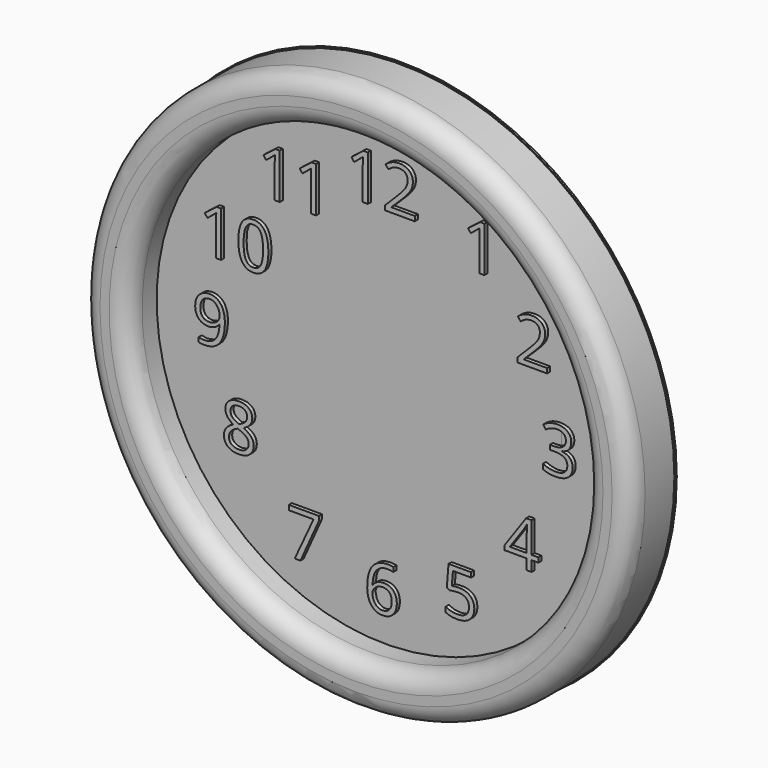
from build123d import *

# Parameters (mm, degrees)
F0_R         = 38.1
F0_R_2       = 31.75
F1_DEPTH     = 7.62
F2_DEPTH     = 2.54
F3_DEPTH     = 2.54
F4_DEPTH     = 2.54
F5_DEPTH     = 2.54
F0_TEXT_SIZE = 8.8194444444
F6_DEPTH     = 3.0734
F7_R         = 2.54
F8_DEPTH     = 2.54
F9_DEPTH     = 2.54
F10_R        = 38.2366779264
F11_DEPTH    = 0.254


# Not quite as in the source:
# - Text() gives the source's letters only with a copy of the font that has no kerning and outlines rounded to 1/6400 em; it was checked with that copy


with BuildPart() as f1:
    # F0 (on Front) → F1 (new body)
    with BuildSketch(Plane.XZ):
        Circle(F0_R)
        Circle(F0_R_2, mode=Mode.SUBTRACT)
    extrude(amount=F1_DEPTH)

    # F7
    f7_edges = [f1.edges().sort_by_distance(p)[0] for p in [
        (-38.1, -7.62, 0),
        (-31.75, -7.62, 0),
    ]]
    fillet(f7_edges, radius=F7_R)


with BuildPart() as f2:
    # F0 (on Front) → F2 (new body)
    with BuildSketch(Plane.XZ):
        with BuildLine():
            add(Edge.make_bspline(
                [(-18.9333114864, 13.2705580962), (-19.256461443, 12.6483738514), (-19.256461443, 11.2744697715)],
                knots=[0, 0, 0, 1, 1, 1], degree=2))
            add(Edge.make_bspline(
                [(-19.256461443, 11.2744697715), (-19.256461443, 9.9005656917), (-18.9333114864, 9.2735583132)],
                knots=[0, 0, 0, 1, 1, 1], degree=2))
            add(Edge.make_bspline(
                [(-18.9333114864, 9.2735583132), (-18.6101615298, 8.6465509347), (-17.9046059742, 8.6465509347)],
                knots=[0, 0, 0, 1, 1, 1], degree=2))
            add(Edge.make_bspline(
                [(-17.9046059742, 8.6465509347), (-17.1894041513, 8.6465509347), (-16.8690102711, 9.2818265424)],
                knots=[0, 0, 0, 1, 1, 1], degree=2))
            add(Edge.make_bspline(
                [(-16.8690102711, 9.2818265424), (-16.5486163909, 9.91710215), (-16.5486163909, 11.2744697715)],
                knots=[0, 0, 0, 1, 1, 1], degree=2))
            add(Edge.make_bspline(
                [(-16.5486163909, 11.2744697715), (-16.5486163909, 12.6304593549), (-16.8690102711, 13.2616008479)],
                knots=[0, 0, 0, 1, 1, 1], degree=2))
            add(Edge.make_bspline(
                [(-16.8690102711, 13.2616008479), (-17.1894041513, 13.892742341), (-17.9046059742, 13.892742341)],
                knots=[0, 0, 0, 1, 1, 1], degree=2))
            add(Edge.make_bspline(
                [(-17.9046059742, 13.892742341), (-18.6101615298, 13.892742341), (-18.9333114864, 13.2705580962)],
                knots=[0, 0, 0, 1, 1, 1], degree=2))
        make_face()
    extrude(amount=F2_DEPTH)


with BuildPart() as f3:
    # F0 (on Front) → F3 (new body)
    with BuildSketch(Plane.XZ):
        with BuildLine():
            Line((17.7058799275, -13.9019929305), (20.0526789726, -13.9019929305))
            Line((20.0526789726, -13.9019929305), (20.0526789726, -11.8087529131))
            add(Edge.make_bspline(
                [(20.0526789726, -11.8087529131), (20.0526789726, -11.1927698402), (20.0967761949, -10.4183123749)],
                knots=[0, 0, 0, 1, 1, 1], degree=2))
            Line((20.0967761949, -10.4183123749), (20.06232524, -10.4183123749))
            add(Edge.make_bspline(
                [(20.06232524, -10.4183123749), (19.8556195108, -10.8317238333), (19.6737184692, -11.1031973576)],
                knots=[0, 0, 0, 1, 1, 1], degree=2))
            Line((19.6737184692, -11.1031973576), (17.7058799275, -13.9019929305))
        make_face()
    extrude(amount=F3_DEPTH)


with BuildPart() as f4:
    # F0 (on Front) → F4 (new body)
    with BuildSketch(Plane.XZ):
        with BuildLine():
            add(Edge.make_bspline(
                [(-23.2508578055, 2.622299725), (-23.5671175712, 2.842096817), (-23.9763949149, 2.842096817)],
                knots=[0, 0, 0, 1, 1, 1], degree=2))
            add(Edge.make_bspline(
                [(-23.9763949149, 2.842096817), (-24.5923779878, 2.842096817), (-24.9279302882, 2.4459108361)],
                knots=[0, 0, 0, 1, 1, 1], degree=2))
            add(Edge.make_bspline(
                [(-24.9279302882, 2.4459108361), (-25.2634825885, 2.0497248552), (-25.2634825885, 1.3427912614)],
                knots=[0, 0, 0, 1, 1, 1], degree=2))
            add(Edge.make_bspline(
                [(-25.2634825885, 1.3427912614), (-25.2634825885, 0.7226740739), (-24.9534239948, 0.3678292389)],
                knots=[0, 0, 0, 1, 1, 1], degree=2))
            add(Edge.make_bspline(
                [(-24.9534239948, 0.3678292389), (-24.643365401, 0.0129844038), (-24.0108458698, 0.0129844038)],
                knots=[0, 0, 0, 1, 1, 1], degree=2))
            add(Edge.make_bspline(
                [(-24.0108458698, 0.0129844038), (-23.6181049844, 0.0129844038), (-23.2887538559, 0.1721478153)],
                knots=[0, 0, 0, 1, 1, 1], degree=2))
            add(Edge.make_bspline(
                [(-23.2887538559, 0.1721478153), (-22.9594027274, 0.3313112267), (-22.7699224757, 0.6069188656)],
                knots=[0, 0, 0, 1, 1, 1], degree=2))
            add(Edge.make_bspline(
                [(-22.7699224757, 0.6069188656), (-22.5804422239, 0.8825265045), (-22.5804422239, 1.1843168691)],
                knots=[0, 0, 0, 1, 1, 1], degree=2))
            add(Edge.make_bspline(
                [(-22.5804422239, 1.1843168691), (-22.5804422239, 1.6363133969), (-22.7575201319, 2.0194080149)],
                knots=[0, 0, 0, 1, 1, 1], degree=2))
            add(Edge.make_bspline(
                [(-22.7575201319, 2.0194080149), (-22.9345980399, 2.402502633), (-23.2508578055, 2.622299725)],
                knots=[0, 0, 0, 1, 1, 1], degree=2))
        make_face()
    extrude(amount=F4_DEPTH)


with BuildPart() as f5:
    # F0 (on Front) → F5 (new body)
    with BuildSketch(Plane.XZ):
        with BuildLine():
            add(Edge.make_bspline(
                [(-0.6952202691, -27.1951703559), (-0.3789605035, -27.4191015625), (0.0261827257, -27.4191015625)],
                knots=[0, 0, 0, 1, 1, 1], degree=2))
            add(Edge.make_bspline(
                [(0.0261827257, -27.4191015625), (0.638031684, -27.4191015625), (0.9756510417, -27.0332508681)],
                knots=[0, 0, 0, 1, 1, 1], degree=2))
            add(Edge.make_bspline(
                [(0.9756510417, -27.0332508681), (1.3132703993, -26.6474001736), (1.3132703993, -25.9197960069)],
                knots=[0, 0, 0, 1, 1, 1], degree=2))
            add(Edge.make_bspline(
                [(1.3132703993, -25.9197960069), (1.3132703993, -25.2955447049), (0.999077691, -24.9379437934)],
                knots=[0, 0, 0, 1, 1, 1], degree=2))
            add(Edge.make_bspline(
                [(0.999077691, -24.9379437934), (0.6848849826, -24.5803428819), (0.0606336806, -24.5803428819)],
                knots=[0, 0, 0, 1, 1, 1], degree=2))
            add(Edge.make_bspline(
                [(0.0606336806, -24.5803428819), (-0.3265950521, -24.5803428819), (-0.6497450087, -24.7401953125)],
                knots=[0, 0, 0, 1, 1, 1], degree=2))
            add(Edge.make_bspline(
                [(-0.6497450087, -24.7401953125), (-0.9728949653, -24.9000477431), (-1.1644422743, -25.1797894965)],
                knots=[0, 0, 0, 1, 1, 1], degree=2))
            add(Edge.make_bspline(
                [(-1.1644422743, -25.1797894965), (-1.3559895833, -25.45953125), (-1.3559895833, -25.7613216146)],
                knots=[0, 0, 0, 1, 1, 1], degree=2))
            add(Edge.make_bspline(
                [(-1.3559895833, -25.7613216146), (-1.3559895833, -26.2050499132), (-1.183734809, -26.5881445313)],
                knots=[0, 0, 0, 1, 1, 1], degree=2))
            add(Edge.make_bspline(
                [(-1.183734809, -26.5881445313), (-1.0114800347, -26.9712391493), (-0.6952202691, -27.1951703559)],
                knots=[0, 0, 0, 1, 1, 1], degree=2))
        make_face()
    extrude(amount=F5_DEPTH)


with BuildPart() as f5b:
    # F0 (on Front) → F5, piece 2 (new body)
    with BuildSketch(Plane.XZ):
        with BuildLine():
            add(Edge.make_bspline(
                [(-20.990759851, -12.3462794049), (-21.2787698337, -12.679764648), (-21.2787698337, -13.1455415577)],
                knots=[0, 0, 0, 1, 1, 1], degree=2))
            add(Edge.make_bspline(
                [(-21.2787698337, -13.1455415577), (-21.2787698337, -13.6623058806), (-20.919790884, -13.9510048824)],
                knots=[0, 0, 0, 1, 1, 1], degree=2))
            add(Edge.make_bspline(
                [(-20.919790884, -13.9510048824), (-20.5608119344, -14.2397038841), (-19.9103779066, -14.2397038841)],
                knots=[0, 0, 0, 1, 1, 1], degree=2))
            add(Edge.make_bspline(
                [(-19.9103779066, -14.2397038841), (-19.268212108, -14.2397038841), (-18.9106111965, -13.9379135195)],
                knots=[0, 0, 0, 1, 1, 1], degree=2))
            add(Edge.make_bspline(
                [(-18.9106111965, -13.9379135195), (-18.553010285, -13.6361231549), (-18.553010285, -13.1110906028)],
                knots=[0, 0, 0, 1, 1, 1], degree=2))
            add(Edge.make_bspline(
                [(-18.553010285, -13.1110906028), (-18.553010285, -12.6935450299), (-18.8892516045, -12.368328016)],
                knots=[0, 0, 0, 1, 1, 1], degree=2))
            add(Edge.make_bspline(
                [(-18.8892516045, -12.368328016), (-19.2254929239, -12.0431110021), (-20.0605840698, -11.737186523)],
                knots=[0, 0, 0, 1, 1, 1], degree=2))
            add(Edge.make_bspline(
                [(-20.0605840698, -11.737186523), (-20.7027498684, -12.0127941619), (-20.990759851, -12.3462794049)],
                knots=[0, 0, 0, 1, 1, 1], degree=2))
        make_face()
    extrude(amount=F5_DEPTH)


with BuildPart() as f5c:
    # F0 (on Front) → F5, piece 3 (new body)
    with BuildSketch(Plane.XZ):
        with BuildLine():
            add(Edge.make_bspline(
                [(-19.0677075507, -9.1850597869), (-19.3798332017, -8.9287446827), (-19.9269143649, -8.9287446827)],
                knots=[0, 0, 0, 1, 1, 1], degree=2))
            add(Edge.make_bspline(
                [(-19.9269143649, -8.9287446827), (-20.4657272989, -8.9287446827), (-20.7716517781, -9.1871268442)],
                knots=[0, 0, 0, 1, 1, 1], degree=2))
            add(Edge.make_bspline(
                [(-20.7716517781, -9.1871268442), (-21.0775762573, -9.4455090056), (-21.0775762573, -9.8768349605)],
                knots=[0, 0, 0, 1, 1, 1], degree=2))
            add(Edge.make_bspline(
                [(-21.0775762573, -9.8768349605), (-21.0775762573, -10.2723319223), (-20.8233282104, -10.5568968094)],
                knots=[0, 0, 0, 1, 1, 1], degree=2))
            add(Edge.make_bspline(
                [(-20.8233282104, -10.5568968094), (-20.5690801635, -10.8414616966), (-19.8841951809, -11.1253375646)],
                knots=[0, 0, 0, 1, 1, 1], degree=2))
            add(Edge.make_bspline(
                [(-19.8841951809, -11.1253375646), (-19.268212108, -10.8676444223), (-19.0118970038, -10.5699881723)],
                knots=[0, 0, 0, 1, 1, 1], degree=2))
            add(Edge.make_bspline(
                [(-19.0118970038, -10.5699881723), (-18.7555818996, -10.2723319223), (-18.7555818996, -9.8768349605)],
                knots=[0, 0, 0, 1, 1, 1], degree=2))
            add(Edge.make_bspline(
                [(-18.7555818996, -9.8768349605), (-18.7555818996, -9.441374891), (-19.0677075507, -9.1850597869)],
                knots=[0, 0, 0, 1, 1, 1], degree=2))
        make_face()
    extrude(amount=F5_DEPTH)


with BuildPart() as f6:
    # F0 (on Front) → F6 (new body)
    with BuildSketch(Plane.XZ):
        with Locations((21.9082459122, -3.175)):
            Text('3', F0_TEXT_SIZE, font='Open Sans', text_align=(TextAlign.LEFT, TextAlign.BOTTOM))
        with Locations((16.8060209865, -15.9993670624)):
            Text('4', F0_TEXT_SIZE, font='Open Sans', text_align=(TextAlign.LEFT, TextAlign.BOTTOM))
        with Locations((8.2414952257, -25.0474884677)):
            Text('5', F0_TEXT_SIZE, font='Open Sans', text_align=(TextAlign.LEFT, TextAlign.BOTTOM))
        with Locations((-2.5920898438, -27.94)):
            Text('6', F0_TEXT_SIZE, font='Open Sans', text_align=(TextAlign.LEFT, TextAlign.BOTTOM))
        with Locations((-13.3781325955, -25.0474884677)):
            Text('7', F0_TEXT_SIZE, font='Open Sans', text_align=(TextAlign.LEFT, TextAlign.BOTTOM))
        with Locations((-22.4335658406, -14.7344195959)):
            Text('8', F0_TEXT_SIZE, font='Open Sans', text_align=(TextAlign.LEFT, TextAlign.BOTTOM))
        with Locations((-26.4265468246, -2.9332612559)):
            Text('9', F0_TEXT_SIZE, font='Open Sans', text_align=(TextAlign.LEFT, TextAlign.BOTTOM))
        with Locations((-25.4617674326, 8.117384268)):
            Text('10', F0_TEXT_SIZE, font='Open Sans', text_align=(TextAlign.LEFT, TextAlign.BOTTOM))
        with Locations((18.3173481208, 8.9695071709)):
            Text('2', F0_TEXT_SIZE, font='Open Sans', text_align=(TextAlign.LEFT, TextAlign.BOTTOM))
        with Locations((11.1048174741, 18.1498409915)):
            Text('1', F0_TEXT_SIZE, font='Open Sans', text_align=(TextAlign.LEFT, TextAlign.BOTTOM))
        with Locations((-5.0918511285, 21.59)):
            Text('12', F0_TEXT_SIZE, font='Open Sans', text_align=(TextAlign.LEFT, TextAlign.BOTTOM))
        with Locations((-17.3156698598, 17.8489641953)):
            Text('11', F0_TEXT_SIZE, font='Open Sans', text_align=(TextAlign.LEFT, TextAlign.BOTTOM))
    extrude(amount=F6_DEPTH)


with BuildPart() as f8:
    # F0 (on Front) → F8 (new body)
    with BuildSketch(Plane.XZ):
        Circle(F0_R_2)
        Polygon((-11.3579286024, -25.0474884677), (-12.1503005642, -25.0474884677), (-9.5416742622, -19.4099342142), (-12.9729893663, -19.4099342142), (-12.9729893663, -18.7512319573), (-8.7837532552, -18.7512319573), (-8.7837532552, -19.3244958462), align=None, mode=Mode.SUBTRACT)
        with BuildLine():
            add(Edge.make_bspline(
                [(-1.5151529948, -27.2923220486), (-2.0877278646, -26.557827691), (-2.0877278646, -25.2486914063)],
                knots=[0, 0, 0, 1, 1, 1], degree=2))
            add(Edge.make_bspline(
                [(-2.0877278646, -25.2486914063), (-2.0877278646, -23.3924739583), (-1.3663248698, -22.4733224826)],
                knots=[0, 0, 0, 1, 1, 1], degree=2))
            add(Edge.make_bspline(
                [(-1.3663248698, -22.4733224826), (-0.644921875, -21.5541710069), (0.7675672743, -21.5541710069)],
                knots=[0, 0, 0, 1, 1, 1], degree=2))
            add(Edge.make_bspline(
                [(0.7675672743, -21.5541710069), (1.2540147569, -21.5541710069), (1.5337565104, -21.6354752604)],
                knots=[0, 0, 0, 1, 1, 1], degree=2))
            Line((1.5337565104, -21.6354752604), (1.5337565104, -22.2514583333))
            add(Edge.make_bspline(
                [(1.5337565104, -22.2514583333), (1.2016493056, -22.1439713542), (0.7758355035, -22.1439713542)],
                knots=[0, 0, 0, 1, 1, 1], degree=2))
            add(Edge.make_bspline(
                [(0.7758355035, -22.1439713542), (-0.2370225694, -22.1439713542), (-0.7710123698, -22.7744238281)],
                knots=[0, 0, 0, 1, 1, 1], degree=2))
            add(Edge.make_bspline(
                [(-0.7710123698, -22.7744238281), (-1.3050021701, -23.4048763021), (-1.3559895833, -24.758109809)],
                knots=[0, 0, 0, 1, 1, 1], degree=2))
            Line((-1.3559895833, -24.758109809), (-1.3050021701, -24.758109809))
            add(Edge.make_bspline(
                [(-1.3050021701, -24.758109809), (-0.8309570313, -24.0167252604), (0.1943033854, -24.0167252604)],
                knots=[0, 0, 0, 1, 1, 1], degree=2))
            add(Edge.make_bspline(
                [(0.1943033854, -24.0167252604), (1.0431749132, -24.0167252604), (1.5316894531, -24.5293554688)],
                knots=[0, 0, 0, 1, 1, 1], degree=2))
            add(Edge.make_bspline(
                [(1.5316894531, -24.5293554688), (2.0202039931, -25.0419856771), (2.0202039931, -25.9197960069)],
                knots=[0, 0, 0, 1, 1, 1], degree=2))
            add(Edge.make_bspline(
                [(2.0202039931, -25.9197960069), (2.0202039931, -26.9023372396), (1.4841471354, -27.4645768229)],
                knots=[0, 0, 0, 1, 1, 1], degree=2))
            add(Edge.make_bspline(
                [(1.4841471354, -27.4645768229), (0.9480902778, -28.0268164063), (0.0344509549, -28.0268164063)],
                knots=[0, 0, 0, 1, 1, 1], degree=2))
            add(Edge.make_bspline(
                [(0.0344509549, -28.0268164063), (-0.942578125, -28.0268164063), (-1.5151529948, -27.2923220486)],
                knots=[0, 0, 0, 1, 1, 1], degree=2))
        make_face(mode=Mode.SUBTRACT)
        with BuildLine():
            add(Edge.make_bspline(
                [(-21.2732576809, -8.7551118702), (-20.7675176635, -8.3485906028), (-19.9186461357, -8.3485906028)],
                knots=[0, 0, 0, 1, 1, 1], degree=2))
            add(Edge.make_bspline(
                [(-19.9186461357, -8.3485906028), (-19.0573722642, -8.3485906028), (-18.5536993041, -8.7489106983)],
                knots=[0, 0, 0, 1, 1, 1], degree=2))
            add(Edge.make_bspline(
                [(-18.5536993041, -8.7489106983), (-18.0500263441, -9.1492307938), (-18.0500263441, -9.8547863494)],
                knots=[0, 0, 0, 1, 1, 1], degree=2))
            add(Edge.make_bspline(
                [(-18.0500263441, -9.8547863494), (-18.0500263441, -10.3205632591), (-18.3380363267, -10.7036578771)],
                knots=[0, 0, 0, 1, 1, 1], degree=2))
            add(Edge.make_bspline(
                [(-18.3380363267, -10.7036578771), (-18.6260463094, -11.0867524952), (-19.2599438788, -11.4009452035)],
                knots=[0, 0, 0, 1, 1, 1], degree=2))
            add(Edge.make_bspline(
                [(-19.2599438788, -11.4009452035), (-18.4937546427, -11.7675033633), (-18.1706046861, -12.169890516)],
                knots=[0, 0, 0, 1, 1, 1], degree=2))
            add(Edge.make_bspline(
                [(-18.1706046861, -12.169890516), (-17.8474547295, -12.5722776688), (-17.8474547295, -13.1028223737)],
                knots=[0, 0, 0, 1, 1, 1], degree=2))
            add(Edge.make_bspline(
                [(-17.8474547295, -13.1028223737), (-17.8474547295, -13.8855480681), (-18.3945358927, -14.3533920351)],
                knots=[0, 0, 0, 1, 1, 1], degree=2))
            add(Edge.make_bspline(
                [(-18.3945358927, -14.3533920351), (-18.9416170559, -14.8212360021), (-19.89246341, -14.8212360021)],
                knots=[0, 0, 0, 1, 1, 1], degree=2))
            add(Edge.make_bspline(
                [(-19.89246341, -14.8212360021), (-20.8998093302, -14.8212360021), (-21.4427563788, -14.3795747608)],
                knots=[0, 0, 0, 1, 1, 1], degree=2))
            add(Edge.make_bspline(
                [(-21.4427563788, -14.3795747608), (-21.9857034274, -13.9379135195), (-21.9857034274, -13.1276270612)],
                knots=[0, 0, 0, 1, 1, 1], degree=2))
            add(Edge.make_bspline(
                [(-21.9857034274, -13.1276270612), (-21.9857034274, -12.0472451167), (-20.6682989135, -11.4436643876)],
                knots=[0, 0, 0, 1, 1, 1], degree=2))
            add(Edge.make_bspline(
                [(-20.6682989135, -11.4436643876), (-21.2622333753, -11.1088011063), (-21.5206155368, -10.7188162973)],
                knots=[0, 0, 0, 1, 1, 1], degree=2))
            add(Edge.make_bspline(
                [(-21.5206155368, -10.7188162973), (-21.7789976982, -10.3288314883), (-21.7789976982, -9.8465181202)],
                knots=[0, 0, 0, 1, 1, 1], degree=2))
            add(Edge.make_bspline(
                [(-21.7789976982, -9.8465181202), (-21.7789976982, -9.1616331376), (-21.2732576809, -8.7551118702)],
                knots=[0, 0, 0, 1, 1, 1], degree=2))
        make_face(mode=Mode.SUBTRACT)
        with BuildLine():
            add(Edge.make_bspline(
                [(9.653984375, -21.300602617), (10.1487000868, -21.201383867), (10.6406597222, -21.201383867)],
                knots=[0, 0, 0, 1, 1, 1], degree=2))
            add(Edge.make_bspline(
                [(10.6406597222, -21.201383867), (11.6356032986, -21.201383867), (12.2061111111, -21.6947215406)],
                knots=[0, 0, 0, 1, 1, 1], degree=2))
            add(Edge.make_bspline(
                [(12.2061111111, -21.6947215406), (12.7766189236, -22.1880592142), (12.7766189236, -23.0451989712)],
                knots=[0, 0, 0, 1, 1, 1], degree=2))
            add(Edge.make_bspline(
                [(12.7766189236, -23.0451989712), (12.7766189236, -24.022228051), (12.1544346788, -24.5782664625)],
                knots=[0, 0, 0, 1, 1, 1], degree=2))
            add(Edge.make_bspline(
                [(12.1544346788, -24.5782664625), (11.532250434, -25.134304874), (10.4380881076, -25.134304874)],
                knots=[0, 0, 0, 1, 1, 1], degree=2))
            add(Edge.make_bspline(
                [(10.4380881076, -25.134304874), (9.3742426215, -25.134304874), (8.8147591146, -24.7939294399)],
                knots=[0, 0, 0, 1, 1, 1], degree=2))
            Line((8.8147591146, -24.7939294399), (8.8147591146, -24.1049103427))
            add(Edge.make_bspline(
                [(8.8147591146, -24.1049103427), (9.115171441, -24.2978356899), (9.5630338542, -24.4080787455)],
                knots=[0, 0, 0, 1, 1, 1], degree=2))
            add(Edge.make_bspline(
                [(9.5630338542, -24.4080787455), (10.0108962674, -24.518321801), (10.4463563368, -24.518321801)],
                knots=[0, 0, 0, 1, 1, 1], degree=2))
            add(Edge.make_bspline(
                [(10.4463563368, -24.518321801), (11.2042773437, -24.518321801), (11.623889974, -24.1607208896)],
                knots=[0, 0, 0, 1, 1, 1], degree=2))
            add(Edge.make_bspline(
                [(11.623889974, -24.1607208896), (12.0435026042, -23.8031199781), (12.0435026042, -23.1265032247)],
                knots=[0, 0, 0, 1, 1, 1], degree=2))
            add(Edge.make_bspline(
                [(12.0435026042, -23.1265032247), (12.0435026042, -21.8090987108), (10.4298198785, -21.8090987108)],
                knots=[0, 0, 0, 1, 1, 1], degree=2))
            add(Edge.make_bspline(
                [(10.4298198785, -21.8090987108), (10.0205425347, -21.8090987108), (9.3356575521, -21.9345001865)],
                knots=[0, 0, 0, 1, 1, 1], degree=2))
            Line((9.3356575521, -21.9345001865), (8.9649652778, -21.697477617))
            Line((8.9649652778, -21.697477617), (9.2019878472, -18.7512319573))
            Line((9.2019878472, -18.7512319573), (12.332890625, -18.7512319573))
            Line((12.332890625, -18.7512319573), (12.332890625, -19.4099342142))
            Line((12.332890625, -19.4099342142), (9.8138368056, -19.4099342142))
            Line((9.8138368056, -19.4099342142), (9.653984375, -21.300602617))
        make_face(mode=Mode.SUBTRACT)
        Polygon((21.6718738511, -13.9019929305), (21.6718738511, -14.5524269583), (20.7375639553, -14.5524269583), (20.7375639553, -15.9993670624), (20.0526789726, -15.9993670624), (20.0526789726, -14.5524269583), (16.9906781046, -14.5524269583), (16.9906781046, -13.9281756562), (19.9796429483, -9.6686595972), (20.7375639553, -9.6686595972), (20.7375639553, -13.9019929305), align=None, mode=Mode.SUBTRACT)
        with BuildLine():
            add(Edge.make_bspline(
                [(23.9022671796, 0.3858506944), (24.2055149995, 0.3858506944), (24.4569275528, 0.4410792403)],
                knots=[0, 0, 0, 0.4120929412, 0.4120929412, 0.4120929412], degree=2))
            Line((24.4569275528, 0.4410792403), (24.4569275528, 2.5961950824))
            add(Edge.make_bspline(
                [(24.4569275528, 2.5961950824), (24.3922299113, 2.6003580729), (24.3239468671, 2.6003580729)],
                knots=[0.8742362732, 0.8742362732, 0.8742362732, 1, 1, 1], degree=2))
            add(Edge.make_bspline(
                [(24.3239468671, 2.6003580729), (23.9105354087, 2.6003580729), (23.5446662681, 2.4880479601)],
                knots=[0, 0, 0, 1, 1, 1], degree=2))
            add(Edge.make_bspline(
                [(23.5446662681, 2.4880479601), (23.1787971275, 2.3757378472), (22.7088861032, 2.0739474826)],
                knots=[0, 0, 0, 1, 1, 1], degree=2))
            Line((22.7088861032, 2.0739474826), (22.3478400962, 2.5562608507))
            add(Edge.make_bspline(
                [(22.3478400962, 2.5562608507), (22.7350688289, 2.8621853299), (23.2408088462, 3.0365071615)],
                knots=[0, 0, 0, 1, 1, 1], degree=2))
            add(Edge.make_bspline(
                [(23.2408088462, 3.0365071615), (23.7465488636, 3.2108289931), (24.3074104087, 3.2108289931)],
                knots=[0, 0, 0, 1, 1, 1], degree=2))
            add(Edge.make_bspline(
                [(24.3074104087, 3.2108289931), (25.223805808, 3.2108289931), (25.7323019018, 2.7912163628)],
                knots=[0, 0, 0, 1, 1, 1], degree=2))
            add(Edge.make_bspline(
                [(25.7323019018, 2.7912163628), (26.2407979955, 2.3716037326), (26.2407979955, 1.6398654514)],
                knots=[0, 0, 0, 1, 1, 1], degree=2))
            add(Edge.make_bspline(
                [(26.2407979955, 1.6398654514), (26.2407979955, 1.0362847222), (25.9024896188, 0.6531901042)],
                knots=[0, 0, 0, 1, 1, 1], degree=2))
            add(Edge.make_bspline(
                [(25.9024896188, 0.6531901042), (25.5641812421, 0.2700954861), (24.9440640546, 0.1405598958)],
                knots=[0, 0, 0, 1, 1, 1], degree=2))
            Line((24.9440640546, 0.1405598958), (24.9440640546, 0.106108941))
            add(Edge.make_bspline(
                [(24.9440640546, 0.106108941), (25.7019850615, 0.0124023437), (26.0678542021, -0.375515408)],
                knots=[0, 0, 0, 1, 1, 1], degree=2))
            add(Edge.make_bspline(
                [(26.0678542021, -0.375515408), (26.4337233427, -0.7634331597), (26.4337233427, -1.3918185764)],
                knots=[0, 0, 0, 1, 1, 1], degree=2))
            add(Edge.make_bspline(
                [(26.4337233427, -1.3918185764), (26.4337233427, -2.2916775174), (25.8094720407, -2.7767469618)],
                knots=[0, 0, 0, 1, 1, 1], degree=2))
            add(Edge.make_bspline(
                [(25.8094720407, -2.7767469618), (25.1852207386, -3.2618164063), (24.0359368844, -3.2618164063)],
                knots=[0, 0, 0, 1, 1, 1], degree=2))
            add(Edge.make_bspline(
                [(24.0359368844, -3.2618164063), (23.5357090198, -3.2618164063), (23.1202305042, -3.1860243056)],
                knots=[0, 0, 0, 1, 1, 1], degree=2))
            add(Edge.make_bspline(
                [(23.1202305042, -3.1860243056), (22.7047519886, -3.1102322049), (22.3133891414, -2.9214409722)],
                knots=[0, 0, 0, 1, 1, 1], degree=2))
            Line((22.3133891414, -2.9214409722), (22.3133891414, -2.2406901042))
            add(Edge.make_bspline(
                [(22.3133891414, -2.2406901042), (22.7226664851, -2.4432617188), (23.1856873184, -2.5486816406)],
                knots=[0, 0, 0, 1, 1, 1], degree=2))
            add(Edge.make_bspline(
                [(23.1856873184, -2.5486816406), (23.6487081518, -2.6541015625), (24.0621196101, -2.6541015625)],
                knots=[0, 0, 0, 1, 1, 1], degree=2))
            add(Edge.make_bspline(
                [(24.0621196101, -2.6541015625), (25.6937168323, -2.6541015625), (25.6937168323, -1.3752821181)],
                knots=[0, 0, 0, 1, 1, 1], degree=2))
            add(Edge.make_bspline(
                [(25.6937168323, -1.3752821181), (25.6937168323, -0.2287543403), (23.8939989504, -0.2287543403)],
                knots=[0, 0, 0, 1, 1, 1], degree=2))
            Line((23.8939989504, -0.2287543403), (23.2738817629, -0.2287543403))
            Line((23.2738817629, -0.2287543403), (23.2738817629, 0.3858506944))
            Line((23.2738817629, 0.3858506944), (23.9022671796, 0.3858506944))
        make_face(mode=Mode.SUBTRACT)
        with BuildLine():
            add(Edge.make_bspline(
                [(-22.1153543333, 2.1634130062), (-21.8569721719, 1.5329605323), (-21.8569721719, 0.6758207753)],
                knots=[0, 0, 0, 1, 1, 1], degree=2))
            add(Edge.make_bspline(
                [(-21.8569721719, 0.6758207753), (-21.8569721719, -3.0200776622), (-24.7164014253, -3.0200776622)],
                knots=[0, 0, 0, 1, 1, 1], degree=2))
            add(Edge.make_bspline(
                [(-24.7164014253, -3.0200776622), (-25.2166292899, -3.0200776622), (-25.5087733871, -2.9332612559)],
                knots=[0, 0, 0, 1, 1, 1], degree=2))
            Line((-25.5087733871, -2.9332612559), (-25.5087733871, -2.317278183))
            add(Edge.make_bspline(
                [(-25.5087733871, -2.317278183), (-25.1642638385, -2.4288992768), (-24.7260476927, -2.4288992768)],
                knots=[0, 0, 0, 1, 1, 1], degree=2))
            add(Edge.make_bspline(
                [(-24.7260476927, -2.4288992768), (-23.6925190469, -2.4288992768), (-23.1647304184, -1.7894895545)],
                knots=[0, 0, 0, 1, 1, 1], degree=2))
            add(Edge.make_bspline(
                [(-23.1647304184, -1.7894895545), (-22.6369417899, -1.1500798323), (-22.5900884913, 0.1714587962)],
                knots=[0, 0, 0, 1, 1, 1], degree=2))
            Line((-22.5900884913, 0.1714587962), (-22.6410759045, 0.1714587962))
            add(Edge.make_bspline(
                [(-22.6410759045, 0.1714587962), (-22.8780984739, -0.1854530962), (-23.2701503403, -0.3728662906)],
                knots=[0, 0, 0, 1, 1, 1], degree=2))
            add(Edge.make_bspline(
                [(-23.2701503403, -0.3728662906), (-23.6622022066, -0.5602794851), (-24.1527838038, -0.5602794851)],
                knots=[0, 0, 0, 1, 1, 1], degree=2))
            add(Edge.make_bspline(
                [(-24.1527838038, -0.5602794851), (-24.9878749496, -0.5602794851), (-25.479145566, -0.0607406396)],
                knots=[0, 0, 0, 1, 1, 1], degree=2))
            add(Edge.make_bspline(
                [(-25.479145566, -0.0607406396), (-25.9704161823, 0.4387982059), (-25.9704161823, 1.3345230323)],
                knots=[0, 0, 0, 1, 1, 1], degree=2))
            add(Edge.make_bspline(
                [(-25.9704161823, 1.3345230323), (-25.9704161823, 2.3156862267), (-25.4212679618, 2.8841269819)],
                knots=[0, 0, 0, 1, 1, 1], degree=2))
            add(Edge.make_bspline(
                [(-25.4212679618, 2.8841269819), (-24.8721197413, 3.4525677371), (-23.9763949149, 3.4525677371)],
                knots=[0, 0, 0, 1, 1, 1], degree=2))
            add(Edge.make_bspline(
                [(-23.9763949149, 3.4525677371), (-23.3342291163, 3.4525677371), (-22.8539828055, 3.1232166087)],
                knots=[0, 0, 0, 1, 1, 1], degree=2))
            add(Edge.make_bspline(
                [(-22.8539828055, 3.1232166087), (-22.3737364948, 2.7938654802), (-22.1153543333, 2.1634130062)],
                knots=[0, 0, 0, 1, 1, 1], degree=2))
        make_face(mode=Mode.SUBTRACT)
        with BuildLine():
            Line((-22.3832301062, 14.4136407785), (-22.3832301062, 8.117384268))
            Line((-22.3832301062, 8.117384268), (-23.0805174326, 8.117384268))
            Line((-23.0805174326, 8.117384268), (-23.0805174326, 12.6042766292))
            add(Edge.make_bspline(
                [(-23.0805174326, 12.6042766292), (-23.0805174326, 13.1651381743), (-23.0460664777, 13.6639880007)],
                knots=[0, 0, 0, 1, 1, 1], degree=2))
            add(Edge.make_bspline(
                [(-23.0460664777, 13.6639880007), (-23.1356389603, 13.5730374799), (-23.2479490732, 13.4745077489)],
                knots=[0, 0, 0, 1, 1, 1], degree=2))
            add(Edge.make_bspline(
                [(-23.2479490732, 13.4745077489), (-23.360259186, 13.375978018), (-24.2725204708, 12.6345934694)],
                knots=[0, 0, 0, 1, 1, 1], degree=2))
            Line((-24.2725204708, 12.6345934694), (-24.6514809742, 13.1251750667))
            Line((-24.6514809742, 13.1251750667), (-22.9854327972, 14.4136407785))
            Line((-22.9854327972, 14.4136407785), (-22.3832301062, 14.4136407785))
        make_face(mode=Mode.SUBTRACT)
        with BuildLine():
            add(Edge.make_bspline(
                [(-16.3474228145, 13.6812134781), (-15.8155000715, 12.8495674278), (-15.8155000715, 11.2744697715)],
                knots=[0, 0, 0, 1, 1, 1], degree=2))
            add(Edge.make_bspline(
                [(-15.8155000715, 11.2744697715), (-15.8155000715, 9.6414945111), (-16.3301973371, 8.8360311864)],
                knots=[0, 0, 0, 1, 1, 1], degree=2))
            add(Edge.make_bspline(
                [(-16.3301973371, 8.8360311864), (-16.8448946027, 8.0305678618), (-17.9046059742, 8.0305678618)],
                knots=[0, 0, 0, 1, 1, 1], degree=2))
            add(Edge.make_bspline(
                [(-17.9046059742, 8.0305678618), (-18.9202201235, 8.0305678618), (-19.4500758093, 8.8553237212)],
                knots=[0, 0, 0, 1, 1, 1], degree=2))
            add(Edge.make_bspline(
                [(-19.4500758093, 8.8553237212), (-19.9799314951, 9.6800795805), (-19.9799314951, 11.2744697715)],
                knots=[0, 0, 0, 1, 1, 1], degree=2))
            add(Edge.make_bspline(
                [(-19.9799314951, 11.2744697715), (-19.9799314951, 12.9184693375), (-19.4673012867, 13.715664433)],
                knots=[0, 0, 0, 1, 1, 1], degree=2))
            add(Edge.make_bspline(
                [(-19.4673012867, 13.715664433), (-18.9546710784, 14.5128595285), (-17.9046059742, 14.5128595285)],
                knots=[0, 0, 0, 1, 1, 1], degree=2))
            add(Edge.make_bspline(
                [(-17.9046059742, 14.5128595285), (-16.8793455576, 14.5128595285), (-16.3474228145, 13.6812134781)],
                knots=[0, 0, 0, 1, 1, 1], degree=2))
        make_face(mode=Mode.SUBTRACT)
        with BuildLine():
            Line((-14.2371325334, 24.1452207057), (-14.2371325334, 17.8489641953))
            Line((-14.2371325334, 17.8489641953), (-14.9344198598, 17.8489641953))
            Line((-14.9344198598, 17.8489641953), (-14.9344198598, 22.3358565564))
            add(Edge.make_bspline(
                [(-14.9344198598, 22.3358565564), (-14.9344198598, 22.8967181015), (-14.899968905, 23.3955679279)],
                knots=[0, 0, 0, 1, 1, 1], degree=2))
            add(Edge.make_bspline(
                [(-14.899968905, 23.3955679279), (-14.9895413876, 23.3046174071), (-15.1018515004, 23.2060876762)],
                knots=[0, 0, 0, 1, 1, 1], degree=2))
            add(Edge.make_bspline(
                [(-15.1018515004, 23.2060876762), (-15.2141616133, 23.1075579453), (-16.126422898, 22.3661733967)],
                knots=[0, 0, 0, 1, 1, 1], degree=2))
            Line((-16.126422898, 22.3661733967), (-16.5053834015, 22.8567549939))
            Line((-16.5053834015, 22.8567549939), (-14.8393352244, 24.1452207057))
            Line((-14.8393352244, 24.1452207057), (-14.2371325334, 24.1452207057))
        make_face(mode=Mode.SUBTRACT)
        with BuildLine():
            Line((-9.19489078, 24.1452207057), (-9.19489078, 17.8489641953))
            Line((-9.19489078, 17.8489641953), (-9.8921781063, 17.8489641953))
            Line((-9.8921781063, 17.8489641953), (-9.8921781063, 22.3358565564))
            add(Edge.make_bspline(
                [(-9.8921781063, 22.3358565564), (-9.8921781063, 22.8967181015), (-9.8577271515, 23.3955679279)],
                knots=[0, 0, 0, 1, 1, 1], degree=2))
            add(Edge.make_bspline(
                [(-9.8577271515, 23.3955679279), (-9.9472996341, 23.3046174071), (-10.059609747, 23.2060876762)],
                knots=[0, 0, 0, 1, 1, 1], degree=2))
            add(Edge.make_bspline(
                [(-10.059609747, 23.2060876762), (-10.1719198598, 23.1075579453), (-11.0841811445, 22.3661733967)],
                knots=[0, 0, 0, 1, 1, 1], degree=2))
            Line((-11.0841811445, 22.3661733967), (-11.463141648, 22.8567549939))
            Line((-11.463141648, 22.8567549939), (-9.7970934709, 24.1452207057))
            Line((-9.7970934709, 24.1452207057), (-9.19489078, 24.1452207057))
        make_face(mode=Mode.SUBTRACT)
        with BuildLine():
            Line((-2.0133138021, 27.8862565104), (-2.0133138021, 21.59))
            Line((-2.0133138021, 21.59), (-2.7106011285, 21.59))
            Line((-2.7106011285, 21.59), (-2.7106011285, 26.0768923611))
            add(Edge.make_bspline(
                [(-2.7106011285, 26.0768923611), (-2.7106011285, 26.6377539063), (-2.6761501736, 27.1366037326)],
                knots=[0, 0, 0, 1, 1, 1], degree=2))
            add(Edge.make_bspline(
                [(-2.6761501736, 27.1366037326), (-2.7657226563, 27.0456532118), (-2.8780327691, 26.9471234809)],
                knots=[0, 0, 0, 1, 1, 1], degree=2))
            add(Edge.make_bspline(
                [(-2.8780327691, 26.9471234809), (-2.9903428819, 26.84859375), (-3.9026041667, 26.1072092014)],
                knots=[0, 0, 0, 1, 1, 1], degree=2))
            Line((-3.9026041667, 26.1072092014), (-4.2815646701, 26.5977907986))
            Line((-4.2815646701, 26.5977907986), (-2.6155164931, 27.8862565104))
            Line((-2.6155164931, 27.8862565104), (-2.0133138021, 27.8862565104))
        make_face(mode=Mode.SUBTRACT)
        with BuildLine():
            Line((22.8869227735, 9.6323435424), (22.8869227735, 8.9695071709))
            Line((22.8869227735, 8.9695071709), (18.7486740756, 8.9695071709))
            Line((18.7486740756, 8.9695071709), (18.7486740756, 9.5854902438))
            Line((18.7486740756, 9.5854902438), (20.4064540235, 11.2515384209))
            add(Edge.make_bspline(
                [(20.4064540235, 11.2515384209), (21.1643750305, 12.0191056952), (21.4055317145, 12.3463897664)],
                knots=[0, 0, 0, 1, 1, 1], degree=2))
            add(Edge.make_bspline(
                [(21.4055317145, 12.3463897664), (21.6466883985, 12.6736738376), (21.7672667405, 12.9837324313)],
                knots=[0, 0, 0, 1, 1, 1], degree=2))
            add(Edge.make_bspline(
                [(21.7672667405, 12.9837324313), (21.8878450826, 13.2937910251), (21.8878450826, 13.6507029174)],
                knots=[0, 0, 0, 1, 1, 1], degree=2))
            add(Edge.make_bspline(
                [(21.8878450826, 13.6507029174), (21.8878450826, 14.1550648966), (21.5819206034, 14.4499650702)],
                knots=[0, 0, 0, 1, 1, 1], degree=2))
            add(Edge.make_bspline(
                [(21.5819206034, 14.4499650702), (21.2759961242, 14.7448652438), (20.7330490756, 14.7448652438)],
                knots=[0, 0, 0, 1, 1, 1], degree=2))
            add(Edge.make_bspline(
                [(20.7330490756, 14.7448652438), (20.3416862284, 14.7448652438), (19.9902864888, 14.6153296536)],
                knots=[0, 0, 0, 1, 1, 1], degree=2))
            add(Edge.make_bspline(
                [(19.9902864888, 14.6153296536), (19.6388867492, 14.4857940633), (19.2089388326, 14.1454186292)],
                knots=[0, 0, 0, 1, 1, 1], degree=2))
            Line((19.2089388326, 14.1454186292), (18.8299783291, 14.6318661119))
            add(Edge.make_bspline(
                [(18.8299783291, 14.6318661119), (19.6995204298, 15.355336164), (20.7247808464, 15.355336164)],
                knots=[0, 0, 0, 1, 1, 1], degree=2))
            add(Edge.make_bspline(
                [(20.7247808464, 15.355336164), (21.6122374437, 15.355336164), (22.1159104037, 14.9012725789)],
                knots=[0, 0, 0, 1, 1, 1], degree=2))
            add(Edge.make_bspline(
                [(22.1159104037, 14.9012725789), (22.6195833638, 14.4472089938), (22.6195833638, 13.6810197577)],
                knots=[0, 0, 0, 1, 1, 1], degree=2))
            add(Edge.make_bspline(
                [(22.6195833638, 13.6810197577), (22.6195833638, 13.0815731431), (22.2833420444, 12.4959069105)],
                knots=[0, 0, 0, 1, 1, 1], degree=2))
            add(Edge.make_bspline(
                [(22.2833420444, 12.4959069105), (21.9471007249, 11.9102406779), (21.026571211, 11.0145158515)],
                knots=[0, 0, 0, 1, 1, 1], degree=2))
            Line((21.026571211, 11.0145158515), (19.6485330166, 9.6667944973))
            Line((19.6485330166, 9.6667944973), (19.6485330166, 9.6323435424))
            Line((19.6485330166, 9.6323435424), (22.8869227735, 9.6323435424))
        make_face(mode=Mode.SUBTRACT)
        with BuildLine():
            Line((4.5199652778, 22.2528363715), (4.5199652778, 21.59))
            Line((4.5199652778, 21.59), (0.3817165799, 21.59))
            Line((0.3817165799, 21.59), (0.3817165799, 22.2059830729))
            Line((0.3817165799, 22.2059830729), (2.0394965278, 23.87203125))
            add(Edge.make_bspline(
                [(2.0394965278, 23.87203125), (2.7974175347, 24.6395985243), (3.0385742188, 24.9668825955)],
                knots=[0, 0, 0, 1, 1, 1], degree=2))
            add(Edge.make_bspline(
                [(3.0385742188, 24.9668825955), (3.2797309028, 25.2941666667), (3.4003092448, 25.6042252604)],
                knots=[0, 0, 0, 1, 1, 1], degree=2))
            add(Edge.make_bspline(
                [(3.4003092448, 25.6042252604), (3.5208875868, 25.9142838542), (3.5208875868, 26.2711957465)],
                knots=[0, 0, 0, 1, 1, 1], degree=2))
            add(Edge.make_bspline(
                [(3.5208875868, 26.2711957465), (3.5208875868, 26.7755577257), (3.2149631076, 27.0704578993)],
                knots=[0, 0, 0, 1, 1, 1], degree=2))
            add(Edge.make_bspline(
                [(3.2149631076, 27.0704578993), (2.9090386285, 27.3653580729), (2.3660915799, 27.3653580729)],
                knots=[0, 0, 0, 1, 1, 1], degree=2))
            add(Edge.make_bspline(
                [(2.3660915799, 27.3653580729), (1.9747287326, 27.3653580729), (1.6233289931, 27.2358224826)],
                knots=[0, 0, 0, 1, 1, 1], degree=2))
            add(Edge.make_bspline(
                [(1.6233289931, 27.2358224826), (1.2719292535, 27.1062868924), (0.8419813368, 26.7659114583)],
                knots=[0, 0, 0, 1, 1, 1], degree=2))
            Line((0.8419813368, 26.7659114583), (0.4630208333, 27.252358941))
            add(Edge.make_bspline(
                [(0.4630208333, 27.252358941), (1.332562934, 27.9758289931), (2.3578233507, 27.9758289931)],
                knots=[0, 0, 0, 1, 1, 1], degree=2))
            add(Edge.make_bspline(
                [(2.3578233507, 27.9758289931), (3.2452799479, 27.9758289931), (3.748952908, 27.521765408)],
                knots=[0, 0, 0, 1, 1, 1], degree=2))
            add(Edge.make_bspline(
                [(3.748952908, 27.521765408), (4.2526258681, 27.0677018229), (4.2526258681, 26.3015125868)],
                knots=[0, 0, 0, 1, 1, 1], degree=2))
            add(Edge.make_bspline(
                [(4.2526258681, 26.3015125868), (4.2526258681, 25.7020659722), (3.9163845486, 25.1163997396)],
                knots=[0, 0, 0, 1, 1, 1], degree=2))
            add(Edge.make_bspline(
                [(3.9163845486, 25.1163997396), (3.5801432292, 24.5307335069), (2.6596137153, 23.6350086806)],
                knots=[0, 0, 0, 1, 1, 1], degree=2))
            Line((2.6596137153, 23.6350086806), (1.2815755208, 22.2872873264))
            Line((1.2815755208, 22.2872873264), (1.2815755208, 22.2528363715))
            Line((1.2815755208, 22.2528363715), (4.5199652778, 22.2528363715))
        make_face(mode=Mode.SUBTRACT)
        with BuildLine():
            Line((14.1833548005, 24.4460975019), (14.1833548005, 18.1498409915))
            Line((14.1833548005, 18.1498409915), (13.4860674741, 18.1498409915))
            Line((13.4860674741, 18.1498409915), (13.4860674741, 22.6367333526))
            add(Edge.make_bspline(
                [(13.4860674741, 22.6367333526), (13.4860674741, 23.1975948978), (13.5205184289, 23.6964447241)],
                knots=[0, 0, 0, 1, 1, 1], degree=2))
            add(Edge.make_bspline(
                [(13.5205184289, 23.6964447241), (13.4309459463, 23.6054942033), (13.3186358335, 23.5069644724)],
                knots=[0, 0, 0, 1, 1, 1], degree=2))
            add(Edge.make_bspline(
                [(13.3186358335, 23.5069644724), (13.2063257206, 23.4084347415), (12.2940644359, 22.6670501929)],
                knots=[0, 0, 0, 1, 1, 1], degree=2))
            Line((12.2940644359, 22.6670501929), (11.9151039324, 23.1576317901))
            Line((11.9151039324, 23.1576317901), (13.5811521095, 24.4460975019))
            Line((13.5811521095, 24.4460975019), (14.1833548005, 24.4460975019))
        make_face(mode=Mode.SUBTRACT)
    extrude(amount=F8_DEPTH)


with BuildPart() as f9:
    # F0 (on Front) → F9 (new body)
    with BuildSketch(Plane.XZ):
        with BuildLine():
            Line((24.4569275528, 2.5961950824), (24.4569275528, 0.4410792403))
            add(Edge.make_bspline(
                [(24.4569275528, 0.4410792403), (24.8156020168, 0.5198703302), (25.0687765112, 0.7110677083)],
                knots=[0.4120929412, 0.4120929412, 0.4120929412, 1, 1, 1], degree=2))
            add(Edge.make_bspline(
                [(25.0687765112, 0.7110677083), (25.4994134469, 1.0362847222), (25.4994134469, 1.6136827257)],
                knots=[0, 0, 0, 1, 1, 1], degree=2))
            add(Edge.make_bspline(
                [(25.4994134469, 1.6136827257), (25.4994134469, 2.0739474826), (25.1831536813, 2.3371527778)],
                knots=[0, 0, 0, 1, 1, 1], degree=2))
            add(Edge.make_bspline(
                [(25.1831536813, 2.3371527778), (24.9066679224, 2.5672563941), (24.4569275528, 2.5961950824)],
                knots=[0, 0, 0, 0.8742362732, 0.8742362732, 0.8742362732], degree=2))
        make_face()
    extrude(amount=F9_DEPTH)


with BuildPart() as f11:
    # F10 (on Front) → F11 (new body)
    with BuildSketch(Plane.XZ):
        Circle(F10_R)
    extrude(amount=-F11_DEPTH)


solid = Compound([f1.part, f2.part, f3.part, f4.part, f5.part, f5b.part, f5c.part, f6.part, f8.part, f9.part, f11.part])
